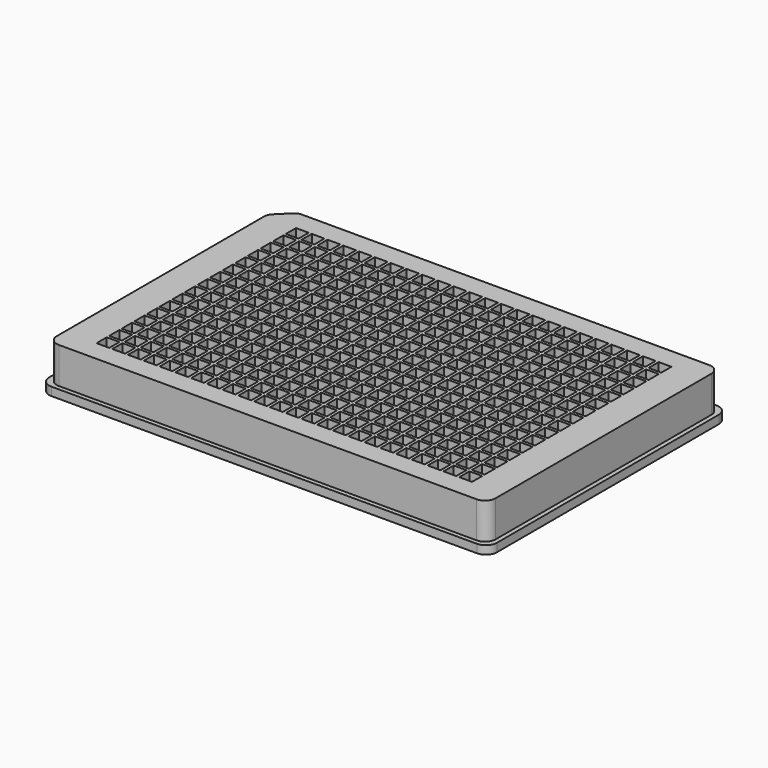
from build123d import *

# Parameters (mm, degrees)
F1_DEPTH = 2.38125
F3_DEPTH = 12.7
F4_W     = 3.63
F4_H     = 3.63
F5_DEPTH = 12.54


# Not quite as in the source:
# - a length typed as a fraction of an inch, garbled in the dataset ("3 / 203.2 mm" for 3/8 in), is restored


with BuildPart() as f1:
    # F0 (on Top) → F1 (new body)
    with BuildSketch(Plane.XY):
        with BuildLine():
            Line((60.7, 42.74), (-60.7, 42.74))
            ThreePointArc((-60.7, 42.74), (-62.9485995642, 41.8085995642), (-63.88, 39.56))
            Line((-63.88, 39.56), (-63.88, -39.56))
            ThreePointArc((-63.88, -39.56), (-62.9485995642, -41.8085995642), (-60.7, -42.74))
            Line((-60.7, -42.74), (60.7, -42.74))
            ThreePointArc((60.7, -42.74), (62.9485995642, -41.8085995642), (63.88, -39.56))
            Line((63.88, -39.56), (63.88, 39.56))
            ThreePointArc((63.88, 39.56), (62.9485995642, 41.8085995642), (60.7, 42.74))
        make_face()
    extrude(amount=F1_DEPTH)

    # F2 (on Top) → F3 (join)
    with BuildSketch(Plane.XY):
        with BuildLine():
            Line((-59.61, -41.47), (59.61, -41.47))
            ThreePointArc((59.61, -41.47), (61.7313203436, -40.5913203436), (62.61, -38.47))
            Line((62.61, -38.47), (62.61, 38.47))
            ThreePointArc((62.61, 38.47), (61.7313203436, 40.5913203436), (59.61, 41.47))
            Line((59.61, 41.47), (-56.5413593129, 41.47))
            ThreePointArc((-56.5413593129, 41.47), (-57.68940961, 41.2416385975), (-58.6626796564, 40.5913203436))
            Line((-58.6626796564, 40.5913203436), (-61.7313203436, 37.5226796564))
            ThreePointArc((-61.7313203436, 37.5226796564), (-62.3816385975, 36.54940961), (-62.61, 35.4013593129))
            Line((-62.61, 35.4013593129), (-62.61, -38.47))
            ThreePointArc((-62.61, -38.47), (-61.7313203436, -40.5913203436), (-59.61, -41.47))
        make_face()
    extrude(amount=F3_DEPTH)

    # F4 (on face) → F5 (cut)
    with BuildSketch(Plane.XY.offset(12.7)):
        with Locations((-51.75, 33.75)):
            Rectangle(F4_W, F4_H)
        with Locations((-51.75, 29.25)):
            Rectangle(F4_W, F4_H)
        with Locations((-51.75, 24.75)):
            Rectangle(F4_W, F4_H)
        with Locations((-51.75, 20.25)):
            Rectangle(F4_W, F4_H)
        with Locations((-51.75, 15.75)):
            Rectangle(F4_W, F4_H)
        with Locations((-51.75, 11.25)):
            Rectangle(F4_W, F4_H)
        with Locations((-51.75, 6.75)):
            Rectangle(F4_W, F4_H)
        with Locations((-51.75, 2.25)):
            Rectangle(F4_W, F4_H)
        with Locations((-51.75, -2.25)):
            Rectangle(F4_W, F4_H)
        with Locations((-51.75, -6.75)):
            Rectangle(F4_W, F4_H)
        with Locations((-51.75, -11.25)):
            Rectangle(F4_W, F4_H)
        with Locations((-51.75, -15.75)):
            Rectangle(F4_W, F4_H)
        with Locations((-51.75, -20.25)):
            Rectangle(F4_W, F4_H)
        with Locations((-51.75, -24.75)):
            Rectangle(F4_W, F4_H)
        with Locations((-51.75, -29.25)):
            Rectangle(F4_W, F4_H)
        with Locations((-51.75, -33.75)):
            Rectangle(F4_W, F4_H)
        with Locations((-47.25, 29.25)):
            Rectangle(F4_W, F4_H)
        with Locations((-47.25, -11.25)):
            Rectangle(F4_W, F4_H)
        with Locations((-47.25, 11.25)):
            Rectangle(F4_W, F4_H)
        with Locations((-47.25, -29.25)):
            Rectangle(F4_W, F4_H)
        with Locations((-47.25, 6.75)):
            Rectangle(F4_W, F4_H)
        with Locations((-47.25, 33.75)):
            Rectangle(F4_W, F4_H)
        with Locations((-47.25, 20.25)):
            Rectangle(F4_W, F4_H)
        with Locations((-47.25, -6.75)):
            Rectangle(F4_W, F4_H)
        with Locations((-47.25, -24.75)):
            Rectangle(F4_W, F4_H)
        with Locations((-47.25, 15.75)):
            Rectangle(F4_W, F4_H)
        with Locations((-47.25, -2.25)):
            Rectangle(F4_W, F4_H)
        with Locations((-47.25, -20.25)):
            Rectangle(F4_W, F4_H)
        with Locations((-47.25, -15.75)):
            Rectangle(F4_W, F4_H)
        with Locations((-47.25, -33.75)):
            Rectangle(F4_W, F4_H)
        with Locations((-47.25, 2.25)):
            Rectangle(F4_W, F4_H)
        with Locations((-47.25, 24.75)):
            Rectangle(F4_W, F4_H)
        with Locations((-42.75, 29.25)):
            Rectangle(F4_W, F4_H)
        with Locations((-42.75, -11.25)):
            Rectangle(F4_W, F4_H)
        with Locations((-42.75, 11.25)):
            Rectangle(F4_W, F4_H)
        with Locations((-42.75, -29.25)):
            Rectangle(F4_W, F4_H)
        with Locations((-42.75, 6.75)):
            Rectangle(F4_W, F4_H)
        with Locations((-42.75, 33.75)):
            Rectangle(F4_W, F4_H)
        with Locations((-42.75, 20.25)):
            Rectangle(F4_W, F4_H)
        with Locations((-42.75, -6.75)):
            Rectangle(F4_W, F4_H)
        with Locations((-42.75, -24.75)):
            Rectangle(F4_W, F4_H)
        with Locations((-42.75, 15.75)):
            Rectangle(F4_W, F4_H)
        with Locations((-42.75, -2.25)):
            Rectangle(F4_W, F4_H)
        with Locations((-42.75, -20.25)):
            Rectangle(F4_W, F4_H)
        with Locations((-42.75, -15.75)):
            Rectangle(F4_W, F4_H)
        with Locations((-42.75, -33.75)):
            Rectangle(F4_W, F4_H)
        with Locations((-42.75, 2.25)):
            Rectangle(F4_W, F4_H)
        with Locations((-42.75, 24.75)):
            Rectangle(F4_W, F4_H)
        with Locations((-38.25, 29.25)):
            Rectangle(F4_W, F4_H)
        with Locations((-38.25, -11.25)):
            Rectangle(F4_W, F4_H)
        with Locations((-38.25, 11.25)):
            Rectangle(F4_W, F4_H)
        with Locations((-38.25, -29.25)):
            Rectangle(F4_W, F4_H)
        with Locations((-38.25, 6.75)):
            Rectangle(F4_W, F4_H)
        with Locations((-38.25, 33.75)):
            Rectangle(F4_W, F4_H)
        with Locations((-38.25, 20.25)):
            Rectangle(F4_W, F4_H)
        with Locations((-38.25, -6.75)):
            Rectangle(F4_W, F4_H)
        with Locations((-38.25, -24.75)):
            Rectangle(F4_W, F4_H)
        with Locations((-38.25, 15.75)):
            Rectangle(F4_W, F4_H)
        with Locations((-38.25, -2.25)):
            Rectangle(F4_W, F4_H)
        with Locations((-38.25, -20.25)):
            Rectangle(F4_W, F4_H)
        with Locations((-38.25, -15.75)):
            Rectangle(F4_W, F4_H)
        with Locations((-38.25, -33.75)):
            Rectangle(F4_W, F4_H)
        with Locations((-38.25, 2.25)):
            Rectangle(F4_W, F4_H)
        with Locations((-38.25, 24.75)):
            Rectangle(F4_W, F4_H)
        with Locations((-33.75, 29.25)):
            Rectangle(F4_W, F4_H)
        with Locations((-33.75, -11.25)):
            Rectangle(F4_W, F4_H)
        with Locations((-33.75, 11.25)):
            Rectangle(F4_W, F4_H)
        with Locations((-33.75, -29.25)):
            Rectangle(F4_W, F4_H)
        with Locations((-33.75, 6.75)):
            Rectangle(F4_W, F4_H)
        with Locations((-33.75, 33.75)):
            Rectangle(F4_W, F4_H)
        with Locations((-33.75, 20.25)):
            Rectangle(F4_W, F4_H)
        with Locations((-33.75, -6.75)):
            Rectangle(F4_W, F4_H)
        with Locations((-33.75, -24.75)):
            Rectangle(F4_W, F4_H)
        with Locations((-33.75, 15.75)):
            Rectangle(F4_W, F4_H)
        with Locations((-33.75, -2.25)):
            Rectangle(F4_W, F4_H)
        with Locations((-33.75, -20.25)):
            Rectangle(F4_W, F4_H)
        with Locations((-33.75, -15.75)):
            Rectangle(F4_W, F4_H)
        with Locations((-33.75, -33.75)):
            Rectangle(F4_W, F4_H)
        with Locations((-33.75, 2.25)):
            Rectangle(F4_W, F4_H)
        with Locations((-33.75, 24.75)):
            Rectangle(F4_W, F4_H)
        with Locations((-29.25, 29.25)):
            Rectangle(F4_W, F4_H)
        with Locations((-29.25, -11.25)):
            Rectangle(F4_W, F4_H)
        with Locations((-29.25, 11.25)):
            Rectangle(F4_W, F4_H)
        with Locations((-29.25, -29.25)):
            Rectangle(F4_W, F4_H)
        with Locations((-29.25, 6.75)):
            Rectangle(F4_W, F4_H)
        with Locations((-29.25, 33.75)):
            Rectangle(F4_W, F4_H)
        with Locations((-29.25, 20.25)):
            Rectangle(F4_W, F4_H)
        with Locations((-29.25, -6.75)):
            Rectangle(F4_W, F4_H)
        with Locations((-29.25, -24.75)):
            Rectangle(F4_W, F4_H)
        with Locations((-29.25, 15.75)):
            Rectangle(F4_W, F4_H)
        with Locations((-29.25, -2.25)):
            Rectangle(F4_W, F4_H)
        with Locations((-29.25, -20.25)):
            Rectangle(F4_W, F4_H)
        with Locations((-29.25, -15.75)):
            Rectangle(F4_W, F4_H)
        with Locations((-29.25, -33.75)):
            Rectangle(F4_W, F4_H)
        with Locations((-29.25, 2.25)):
            Rectangle(F4_W, F4_H)
        with Locations((-29.25, 24.75)):
            Rectangle(F4_W, F4_H)
        with Locations((-24.75, 29.25)):
            Rectangle(F4_W, F4_H)
        with Locations((-24.75, -11.25)):
            Rectangle(F4_W, F4_H)
        with Locations((-24.75, 11.25)):
            Rectangle(F4_W, F4_H)
        with Locations((-24.75, -29.25)):
            Rectangle(F4_W, F4_H)
        with Locations((-24.75, 6.75)):
            Rectangle(F4_W, F4_H)
        with Locations((-24.75, 33.75)):
            Rectangle(F4_W, F4_H)
        with Locations((-24.75, 20.25)):
            Rectangle(F4_W, F4_H)
        with Locations((-24.75, -6.75)):
            Rectangle(F4_W, F4_H)
        with Locations((-24.75, -24.75)):
            Rectangle(F4_W, F4_H)
        with Locations((-24.75, 15.75)):
            Rectangle(F4_W, F4_H)
        with Locations((-24.75, -2.25)):
            Rectangle(F4_W, F4_H)
        with Locations((-24.75, -20.25)):
            Rectangle(F4_W, F4_H)
        with Locations((-24.75, -15.75)):
            Rectangle(F4_W, F4_H)
        with Locations((-24.75, -33.75)):
            Rectangle(F4_W, F4_H)
        with Locations((-24.75, 2.25)):
            Rectangle(F4_W, F4_H)
        with Locations((-24.75, 24.75)):
            Rectangle(F4_W, F4_H)
        with Locations((-20.25, 29.25)):
            Rectangle(F4_W, F4_H)
        with Locations((-20.25, -11.25)):
            Rectangle(F4_W, F4_H)
        with Locations((-20.25, 11.25)):
            Rectangle(F4_W, F4_H)
        with Locations((-20.25, -29.25)):
            Rectangle(F4_W, F4_H)
        with Locations((-20.25, 6.75)):
            Rectangle(F4_W, F4_H)
        with Locations((-20.25, 33.75)):
            Rectangle(F4_W, F4_H)
        with Locations((-20.25, 20.25)):
            Rectangle(F4_W, F4_H)
        with Locations((-20.25, -6.75)):
            Rectangle(F4_W, F4_H)
        with Locations((-20.25, -24.75)):
            Rectangle(F4_W, F4_H)
        with Locations((-20.25, 15.75)):
            Rectangle(F4_W, F4_H)
        with Locations((-20.25, -2.25)):
            Rectangle(F4_W, F4_H)
        with Locations((-20.25, -20.25)):
            Rectangle(F4_W, F4_H)
        with Locations((-20.25, -15.75)):
            Rectangle(F4_W, F4_H)
        with Locations((-20.25, -33.75)):
            Rectangle(F4_W, F4_H)
        with Locations((-20.25, 2.25)):
            Rectangle(F4_W, F4_H)
        with Locations((-20.25, 24.75)):
            Rectangle(F4_W, F4_H)
        with Locations((-15.75, 29.25)):
            Rectangle(F4_W, F4_H)
        with Locations((-15.75, -11.25)):
            Rectangle(F4_W, F4_H)
        with Locations((-15.75, 11.25)):
            Rectangle(F4_W, F4_H)
        with Locations((-15.75, -29.25)):
            Rectangle(F4_W, F4_H)
        with Locations((-15.75, 6.75)):
            Rectangle(F4_W, F4_H)
        with Locations((-15.75, 33.75)):
            Rectangle(F4_W, F4_H)
        with Locations((-15.75, 20.25)):
            Rectangle(F4_W, F4_H)
        with Locations((-15.75, -6.75)):
            Rectangle(F4_W, F4_H)
        with Locations((-15.75, -24.75)):
            Rectangle(F4_W, F4_H)
        with Locations((-15.75, 15.75)):
            Rectangle(F4_W, F4_H)
        with Locations((-15.75, -2.25)):
            Rectangle(F4_W, F4_H)
        with Locations((-15.75, -20.25)):
            Rectangle(F4_W, F4_H)
        with Locations((-15.75, -15.75)):
            Rectangle(F4_W, F4_H)
        with Locations((-15.75, -33.75)):
            Rectangle(F4_W, F4_H)
        with Locations((-15.75, 2.25)):
            Rectangle(F4_W, F4_H)
        with Locations((-15.75, 24.75)):
            Rectangle(F4_W, F4_H)
        with Locations((-11.25, 29.25)):
            Rectangle(F4_W, F4_H)
        with Locations((-11.25, -11.25)):
            Rectangle(F4_W, F4_H)
        with Locations((-11.25, 11.25)):
            Rectangle(F4_W, F4_H)
        with Locations((-11.25, -29.25)):
            Rectangle(F4_W, F4_H)
        with Locations((-11.25, 6.75)):
            Rectangle(F4_W, F4_H)
        with Locations((-11.25, 33.75)):
            Rectangle(F4_W, F4_H)
        with Locations((-11.25, 20.25)):
            Rectangle(F4_W, F4_H)
        with Locations((-11.25, -6.75)):
            Rectangle(F4_W, F4_H)
        with Locations((-11.25, -24.75)):
            Rectangle(F4_W, F4_H)
        with Locations((-11.25, 15.75)):
            Rectangle(F4_W, F4_H)
        with Locations((-11.25, -2.25)):
            Rectangle(F4_W, F4_H)
        with Locations((-11.25, -20.25)):
            Rectangle(F4_W, F4_H)
        with Locations((-11.25, -15.75)):
            Rectangle(F4_W, F4_H)
        with Locations((-11.25, -33.75)):
            Rectangle(F4_W, F4_H)
        with Locations((-11.25, 2.25)):
            Rectangle(F4_W, F4_H)
        with Locations((-11.25, 24.75)):
            Rectangle(F4_W, F4_H)
        with Locations((-6.75, 29.25)):
            Rectangle(F4_W, F4_H)
        with Locations((-6.75, -11.25)):
            Rectangle(F4_W, F4_H)
        with Locations((-6.75, 11.25)):
            Rectangle(F4_W, F4_H)
        with Locations((-6.75, -29.25)):
            Rectangle(F4_W, F4_H)
        with Locations((-6.75, 6.75)):
            Rectangle(F4_W, F4_H)
        with Locations((-6.75, 33.75)):
            Rectangle(F4_W, F4_H)
        with Locations((-6.75, 20.25)):
            Rectangle(F4_W, F4_H)
        with Locations((-6.75, -6.75)):
            Rectangle(F4_W, F4_H)
        with Locations((-6.75, -24.75)):
            Rectangle(F4_W, F4_H)
        with Locations((-6.75, 15.75)):
            Rectangle(F4_W, F4_H)
        with Locations((-6.75, -2.25)):
            Rectangle(F4_W, F4_H)
        with Locations((-6.75, -20.25)):
            Rectangle(F4_W, F4_H)
        with Locations((-6.75, -15.75)):
            Rectangle(F4_W, F4_H)
        with Locations((-6.75, -33.75)):
            Rectangle(F4_W, F4_H)
        with Locations((-6.75, 2.25)):
            Rectangle(F4_W, F4_H)
        with Locations((-6.75, 24.75)):
            Rectangle(F4_W, F4_H)
        with Locations((-2.25, 29.25)):
            Rectangle(F4_W, F4_H)
        with Locations((-2.25, -11.25)):
            Rectangle(F4_W, F4_H)
        with Locations((-2.25, 11.25)):
            Rectangle(F4_W, F4_H)
        with Locations((-2.25, -29.25)):
            Rectangle(F4_W, F4_H)
        with Locations((-2.25, 6.75)):
            Rectangle(F4_W, F4_H)
        with Locations((-2.25, 33.75)):
            Rectangle(F4_W, F4_H)
        with Locations((-2.25, 20.25)):
            Rectangle(F4_W, F4_H)
        with Locations((-2.25, -6.75)):
            Rectangle(F4_W, F4_H)
        with Locations((-2.25, -24.75)):
            Rectangle(F4_W, F4_H)
        with Locations((-2.25, 15.75)):
            Rectangle(F4_W, F4_H)
        with Locations((-2.25, -2.25)):
            Rectangle(F4_W, F4_H)
        with Locations((-2.25, -20.25)):
            Rectangle(F4_W, F4_H)
        with Locations((-2.25, -15.75)):
            Rectangle(F4_W, F4_H)
        with Locations((-2.25, -33.75)):
            Rectangle(F4_W, F4_H)
        with Locations((-2.25, 2.25)):
            Rectangle(F4_W, F4_H)
        with Locations((-2.25, 24.75)):
            Rectangle(F4_W, F4_H)
        with Locations((2.25, 29.25)):
            Rectangle(F4_W, F4_H)
        with Locations((2.25, -11.25)):
            Rectangle(F4_W, F4_H)
        with Locations((2.25, 11.25)):
            Rectangle(F4_W, F4_H)
        with Locations((2.25, -29.25)):
            Rectangle(F4_W, F4_H)
        with Locations((2.25, 6.75)):
            Rectangle(F4_W, F4_H)
        with Locations((2.25, 33.75)):
            Rectangle(F4_W, F4_H)
        with Locations((2.25, 20.25)):
            Rectangle(F4_W, F4_H)
        with Locations((2.25, -6.75)):
            Rectangle(F4_W, F4_H)
        with Locations((2.25, -24.75)):
            Rectangle(F4_W, F4_H)
        with Locations((2.25, 15.75)):
            Rectangle(F4_W, F4_H)
        with Locations((2.25, -2.25)):
            Rectangle(F4_W, F4_H)
        with Locations((2.25, -20.25)):
            Rectangle(F4_W, F4_H)
        with Locations((2.25, -15.75)):
            Rectangle(F4_W, F4_H)
        with Locations((2.25, -33.75)):
            Rectangle(F4_W, F4_H)
        with Locations((2.25, 2.25)):
            Rectangle(F4_W, F4_H)
        with Locations((2.25, 24.75)):
            Rectangle(F4_W, F4_H)
        with Locations((6.75, 29.25)):
            Rectangle(F4_W, F4_H)
        with Locations((6.75, -11.25)):
            Rectangle(F4_W, F4_H)
        with Locations((6.75, 11.25)):
            Rectangle(F4_W, F4_H)
        with Locations((6.75, -29.25)):
            Rectangle(F4_W, F4_H)
        with Locations((6.75, 6.75)):
            Rectangle(F4_W, F4_H)
        with Locations((6.75, 33.75)):
            Rectangle(F4_W, F4_H)
        with Locations((6.75, 20.25)):
            Rectangle(F4_W, F4_H)
        with Locations((6.75, -6.75)):
            Rectangle(F4_W, F4_H)
        with Locations((6.75, -24.75)):
            Rectangle(F4_W, F4_H)
        with Locations((6.75, 15.75)):
            Rectangle(F4_W, F4_H)
        with Locations((6.75, -2.25)):
            Rectangle(F4_W, F4_H)
        with Locations((6.75, -20.25)):
            Rectangle(F4_W, F4_H)
        with Locations((6.75, -15.75)):
            Rectangle(F4_W, F4_H)
        with Locations((6.75, -33.75)):
            Rectangle(F4_W, F4_H)
        with Locations((6.75, 2.25)):
            Rectangle(F4_W, F4_H)
        with Locations((6.75, 24.75)):
            Rectangle(F4_W, F4_H)
        with Locations((11.25, 29.25)):
            Rectangle(F4_W, F4_H)
        with Locations((11.25, -11.25)):
            Rectangle(F4_W, F4_H)
        with Locations((11.25, 11.25)):
            Rectangle(F4_W, F4_H)
        with Locations((11.25, -29.25)):
            Rectangle(F4_W, F4_H)
        with Locations((11.25, 6.75)):
            Rectangle(F4_W, F4_H)
        with Locations((11.25, 33.75)):
            Rectangle(F4_W, F4_H)
        with Locations((11.25, 20.25)):
            Rectangle(F4_W, F4_H)
        with Locations((11.25, -6.75)):
            Rectangle(F4_W, F4_H)
        with Locations((11.25, -24.75)):
            Rectangle(F4_W, F4_H)
        with Locations((11.25, 15.75)):
            Rectangle(F4_W, F4_H)
        with Locations((11.25, -2.25)):
            Rectangle(F4_W, F4_H)
        with Locations((11.25, -20.25)):
            Rectangle(F4_W, F4_H)
        with Locations((11.25, -15.75)):
            Rectangle(F4_W, F4_H)
        with Locations((11.25, -33.75)):
            Rectangle(F4_W, F4_H)
        with Locations((11.25, 2.25)):
            Rectangle(F4_W, F4_H)
        with Locations((11.25, 24.75)):
            Rectangle(F4_W, F4_H)
        with Locations((15.75, 29.25)):
            Rectangle(F4_W, F4_H)
        with Locations((15.75, -11.25)):
            Rectangle(F4_W, F4_H)
        with Locations((15.75, 11.25)):
            Rectangle(F4_W, F4_H)
        with Locations((15.75, -29.25)):
            Rectangle(F4_W, F4_H)
        with Locations((15.75, 6.75)):
            Rectangle(F4_W, F4_H)
        with Locations((15.75, 33.75)):
            Rectangle(F4_W, F4_H)
        with Locations((15.75, 20.25)):
            Rectangle(F4_W, F4_H)
        with Locations((15.75, -6.75)):
            Rectangle(F4_W, F4_H)
        with Locations((15.75, -24.75)):
            Rectangle(F4_W, F4_H)
        with Locations((15.75, 15.75)):
            Rectangle(F4_W, F4_H)
        with Locations((15.75, -2.25)):
            Rectangle(F4_W, F4_H)
        with Locations((15.75, -20.25)):
            Rectangle(F4_W, F4_H)
        with Locations((15.75, -15.75)):
            Rectangle(F4_W, F4_H)
        with Locations((15.75, -33.75)):
            Rectangle(F4_W, F4_H)
        with Locations((15.75, 2.25)):
            Rectangle(F4_W, F4_H)
        with Locations((15.75, 24.75)):
            Rectangle(F4_W, F4_H)
        with Locations((20.25, 29.25)):
            Rectangle(F4_W, F4_H)
        with Locations((20.25, -11.25)):
            Rectangle(F4_W, F4_H)
        with Locations((20.25, 11.25)):
            Rectangle(F4_W, F4_H)
        with Locations((20.25, -29.25)):
            Rectangle(F4_W, F4_H)
        with Locations((20.25, 6.75)):
            Rectangle(F4_W, F4_H)
        with Locations((20.25, 33.75)):
            Rectangle(F4_W, F4_H)
        with Locations((20.25, 20.25)):
            Rectangle(F4_W, F4_H)
        with Locations((20.25, -6.75)):
            Rectangle(F4_W, F4_H)
        with Locations((20.25, -24.75)):
            Rectangle(F4_W, F4_H)
        with Locations((20.25, 15.75)):
            Rectangle(F4_W, F4_H)
        with Locations((20.25, -2.25)):
            Rectangle(F4_W, F4_H)
        with Locations((20.25, -20.25)):
            Rectangle(F4_W, F4_H)
        with Locations((20.25, -15.75)):
            Rectangle(F4_W, F4_H)
        with Locations((20.25, -33.75)):
            Rectangle(F4_W, F4_H)
        with Locations((20.25, 2.25)):
            Rectangle(F4_W, F4_H)
        with Locations((20.25, 24.75)):
            Rectangle(F4_W, F4_H)
        with Locations((24.75, 29.25)):
            Rectangle(F4_W, F4_H)
        with Locations((24.75, -11.25)):
            Rectangle(F4_W, F4_H)
        with Locations((24.75, 11.25)):
            Rectangle(F4_W, F4_H)
        with Locations((24.75, -29.25)):
            Rectangle(F4_W, F4_H)
        with Locations((24.75, 6.75)):
            Rectangle(F4_W, F4_H)
        with Locations((24.75, 33.75)):
            Rectangle(F4_W, F4_H)
        with Locations((24.75, 20.25)):
            Rectangle(F4_W, F4_H)
        with Locations((24.75, -6.75)):
            Rectangle(F4_W, F4_H)
        with Locations((24.75, -24.75)):
            Rectangle(F4_W, F4_H)
        with Locations((24.75, 15.75)):
            Rectangle(F4_W, F4_H)
        with Locations((24.75, -2.25)):
            Rectangle(F4_W, F4_H)
        with Locations((24.75, -20.25)):
            Rectangle(F4_W, F4_H)
        with Locations((24.75, -15.75)):
            Rectangle(F4_W, F4_H)
        with Locations((24.75, -33.75)):
            Rectangle(F4_W, F4_H)
        with Locations((24.75, 2.25)):
            Rectangle(F4_W, F4_H)
        with Locations((24.75, 24.75)):
            Rectangle(F4_W, F4_H)
        with Locations((29.25, 29.25)):
            Rectangle(F4_W, F4_H)
        with Locations((29.25, -11.25)):
            Rectangle(F4_W, F4_H)
        with Locations((29.25, 11.25)):
            Rectangle(F4_W, F4_H)
        with Locations((29.25, -29.25)):
            Rectangle(F4_W, F4_H)
        with Locations((29.25, 6.75)):
            Rectangle(F4_W, F4_H)
        with Locations((29.25, 33.75)):
            Rectangle(F4_W, F4_H)
        with Locations((29.25, 20.25)):
            Rectangle(F4_W, F4_H)
        with Locations((29.25, -6.75)):
            Rectangle(F4_W, F4_H)
        with Locations((29.25, -24.75)):
            Rectangle(F4_W, F4_H)
        with Locations((29.25, 15.75)):
            Rectangle(F4_W, F4_H)
        with Locations((29.25, -2.25)):
            Rectangle(F4_W, F4_H)
        with Locations((29.25, -20.25)):
            Rectangle(F4_W, F4_H)
        with Locations((29.25, -15.75)):
            Rectangle(F4_W, F4_H)
        with Locations((29.25, -33.75)):
            Rectangle(F4_W, F4_H)
        with Locations((29.25, 2.25)):
            Rectangle(F4_W, F4_H)
        with Locations((29.25, 24.75)):
            Rectangle(F4_W, F4_H)
        with Locations((33.75, 29.25)):
            Rectangle(F4_W, F4_H)
        with Locations((33.75, -11.25)):
            Rectangle(F4_W, F4_H)
        with Locations((33.75, 11.25)):
            Rectangle(F4_W, F4_H)
        with Locations((33.75, -29.25)):
            Rectangle(F4_W, F4_H)
        with Locations((33.75, 6.75)):
            Rectangle(F4_W, F4_H)
        with Locations((33.75, 33.75)):
            Rectangle(F4_W, F4_H)
        with Locations((33.75, 20.25)):
            Rectangle(F4_W, F4_H)
        with Locations((33.75, -6.75)):
            Rectangle(F4_W, F4_H)
        with Locations((33.75, -24.75)):
            Rectangle(F4_W, F4_H)
        with Locations((33.75, 15.75)):
            Rectangle(F4_W, F4_H)
        with Locations((33.75, -2.25)):
            Rectangle(F4_W, F4_H)
        with Locations((33.75, -20.25)):
            Rectangle(F4_W, F4_H)
        with Locations((33.75, -15.75)):
            Rectangle(F4_W, F4_H)
        with Locations((33.75, -33.75)):
            Rectangle(F4_W, F4_H)
        with Locations((33.75, 2.25)):
            Rectangle(F4_W, F4_H)
        with Locations((33.75, 24.75)):
            Rectangle(F4_W, F4_H)
        with Locations((38.25, 29.25)):
            Rectangle(F4_W, F4_H)
        with Locations((38.25, -11.25)):
            Rectangle(F4_W, F4_H)
        with Locations((38.25, 11.25)):
            Rectangle(F4_W, F4_H)
        with Locations((38.25, -29.25)):
            Rectangle(F4_W, F4_H)
        with Locations((38.25, 6.75)):
            Rectangle(F4_W, F4_H)
        with Locations((38.25, 33.75)):
            Rectangle(F4_W, F4_H)
        with Locations((38.25, 20.25)):
            Rectangle(F4_W, F4_H)
        with Locations((38.25, -6.75)):
            Rectangle(F4_W, F4_H)
        with Locations((38.25, -24.75)):
            Rectangle(F4_W, F4_H)
        with Locations((38.25, 15.75)):
            Rectangle(F4_W, F4_H)
        with Locations((38.25, -2.25)):
            Rectangle(F4_W, F4_H)
        with Locations((38.25, -20.25)):
            Rectangle(F4_W, F4_H)
        with Locations((38.25, -15.75)):
            Rectangle(F4_W, F4_H)
        with Locations((38.25, -33.75)):
            Rectangle(F4_W, F4_H)
        with Locations((38.25, 2.25)):
            Rectangle(F4_W, F4_H)
        with Locations((38.25, 24.75)):
            Rectangle(F4_W, F4_H)
        with Locations((42.75, 29.25)):
            Rectangle(F4_W, F4_H)
        with Locations((42.75, -11.25)):
            Rectangle(F4_W, F4_H)
        with Locations((42.75, 11.25)):
            Rectangle(F4_W, F4_H)
        with Locations((42.75, -29.25)):
            Rectangle(F4_W, F4_H)
        with Locations((42.75, 6.75)):
            Rectangle(F4_W, F4_H)
        with Locations((42.75, 33.75)):
            Rectangle(F4_W, F4_H)
        with Locations((42.75, 20.25)):
            Rectangle(F4_W, F4_H)
        with Locations((42.75, -6.75)):
            Rectangle(F4_W, F4_H)
        with Locations((42.75, -24.75)):
            Rectangle(F4_W, F4_H)
        with Locations((42.75, 15.75)):
            Rectangle(F4_W, F4_H)
        with Locations((42.75, -2.25)):
            Rectangle(F4_W, F4_H)
        with Locations((42.75, -20.25)):
            Rectangle(F4_W, F4_H)
        with Locations((42.75, -15.75)):
            Rectangle(F4_W, F4_H)
        with Locations((42.75, -33.75)):
            Rectangle(F4_W, F4_H)
        with Locations((42.75, 2.25)):
            Rectangle(F4_W, F4_H)
        with Locations((42.75, 24.75)):
            Rectangle(F4_W, F4_H)
        with Locations((47.25, 29.25)):
            Rectangle(F4_W, F4_H)
        with Locations((47.25, -11.25)):
            Rectangle(F4_W, F4_H)
        with Locations((47.25, 11.25)):
            Rectangle(F4_W, F4_H)
        with Locations((47.25, -29.25)):
            Rectangle(F4_W, F4_H)
        with Locations((47.25, 6.75)):
            Rectangle(F4_W, F4_H)
        with Locations((47.25, 33.75)):
            Rectangle(F4_W, F4_H)
        with Locations((47.25, 20.25)):
            Rectangle(F4_W, F4_H)
        with Locations((47.25, -6.75)):
            Rectangle(F4_W, F4_H)
        with Locations((47.25, -24.75)):
            Rectangle(F4_W, F4_H)
        with Locations((47.25, 15.75)):
            Rectangle(F4_W, F4_H)
        with Locations((47.25, -2.25)):
            Rectangle(F4_W, F4_H)
        with Locations((47.25, -20.25)):
            Rectangle(F4_W, F4_H)
        with Locations((47.25, -15.75)):
            Rectangle(F4_W, F4_H)
        with Locations((47.25, -33.75)):
            Rectangle(F4_W, F4_H)
        with Locations((47.25, 2.25)):
            Rectangle(F4_W, F4_H)
        with Locations((47.25, 24.75)):
            Rectangle(F4_W, F4_H)
        with Locations((51.75, 29.25)):
            Rectangle(F4_W, F4_H)
        with Locations((51.75, -11.25)):
            Rectangle(F4_W, F4_H)
        with Locations((51.75, 11.25)):
            Rectangle(F4_W, F4_H)
        with Locations((51.75, -29.25)):
            Rectangle(F4_W, F4_H)
        with Locations((51.75, 6.75)):
            Rectangle(F4_W, F4_H)
        with Locations((51.75, 33.75)):
            Rectangle(F4_W, F4_H)
        with Locations((51.75, 20.25)):
            Rectangle(F4_W, F4_H)
        with Locations((51.75, -6.75)):
            Rectangle(F4_W, F4_H)
        with Locations((51.75, -24.75)):
            Rectangle(F4_W, F4_H)
        with Locations((51.75, 15.75)):
            Rectangle(F4_W, F4_H)
        with Locations((51.75, -2.25)):
            Rectangle(F4_W, F4_H)
        with Locations((51.75, -20.25)):
            Rectangle(F4_W, F4_H)
        with Locations((51.75, -15.75)):
            Rectangle(F4_W, F4_H)
        with Locations((51.75, -33.75)):
            Rectangle(F4_W, F4_H)
        with Locations((51.75, 2.25)):
            Rectangle(F4_W, F4_H)
        with Locations((51.75, 24.75)):
            Rectangle(F4_W, F4_H)
    extrude(amount=-F5_DEPTH, mode=Mode.SUBTRACT)


solid = f1.part
